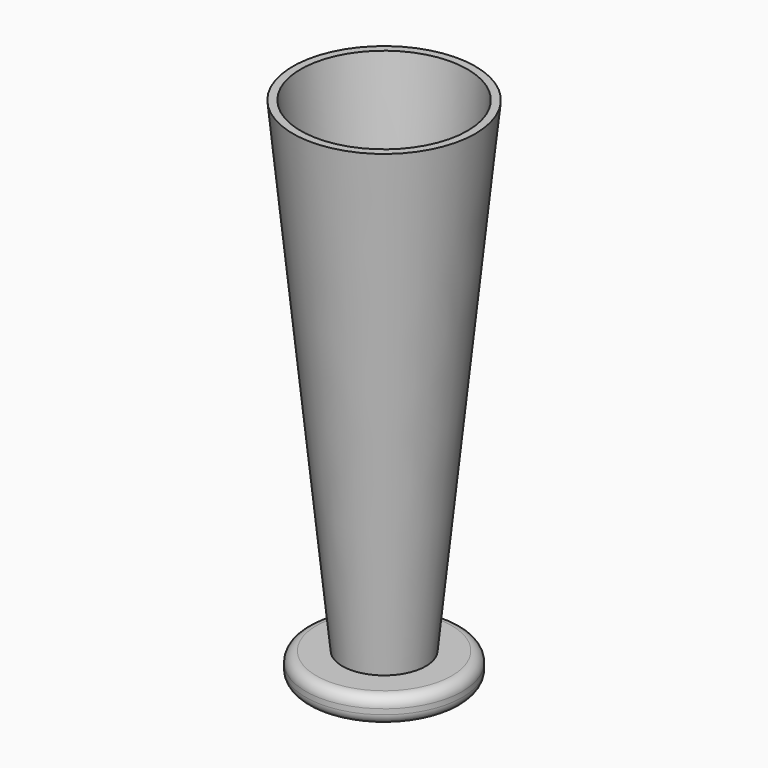
from build123d import *

# Parameters (mm, degrees)
F0_R     = 9.525
F2_R     = 22.225
F6_R     = 19.05
F7_DEPTH = 6.35
F5_R     = 7.62
F4_R     = 20.32
F9_R     = 2.54


with BuildPart() as f3:
    # F0 (on Top) → F3 section 0
    with BuildSketch(Plane.XY):
        Circle(F0_R)
    # F2 (on offset) → F3 section 1
    with BuildSketch(Plane.XY.offset(124.46)):
        Circle(F2_R)
    loft()

    # F6 (on Top) → F7 (join)
    with BuildSketch(Plane.XY):
        Circle(F6_R)
    extrude(amount=F7_DEPTH)

    # F5 (on face) → F8 section 0
    with BuildSketch(Plane(origin=(0, 0, 0), x_dir=(1, 0, 0), z_dir=(0, 0, -1))):
        Circle(F5_R)
    # F4 (on face) → F8 section 1
    with BuildSketch(Plane.XY.offset(124.46)):
        Circle(F4_R)
    loft(mode=Mode.SUBTRACT)

    # F9
    f9_edges = [f3.edges().sort_by_distance(p)[0] for p in [
        (-19.05, 0, 6.35),
        (-19.05, 0, 0),
    ]]
    fillet(f9_edges, radius=F9_R)


solid = f3.part
